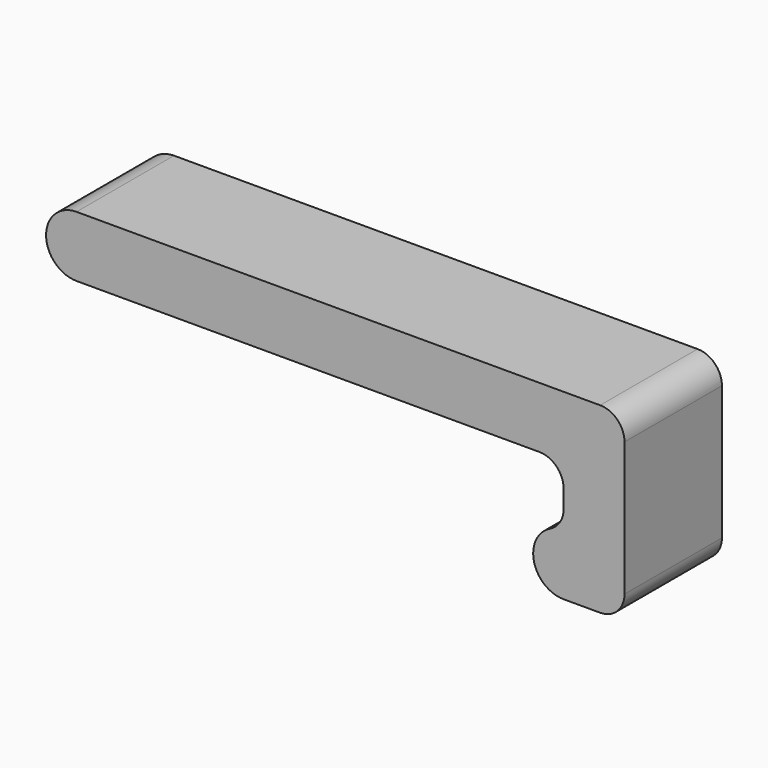
from build123d import *

# Parameters (mm, degrees)
F1_DEPTH = 20
F2_R     = 2.5
F3_DEPTH = 2
F4_R     = 0.99999


# Not quite as in the source:
# - a fillet or chamfer is up to 0.001 mm smaller than in the source, because OpenCascade refuses the exact size


with BuildPart() as f1:
    # F0 (on Front) → F1 (new body)
    with BuildSketch(Plane.XZ):
        with BuildLine():
            ThreePointArc((-42.5, 10), (-47.5, 5), (-42.5, 0))
            Line((-42.5, 0), (33.5, 0))
            ThreePointArc((33.5, 0), (36.3284271247, -1.1715728753), (37.5, -4))
            Line((37.5, -4), (37.5, -6.9377422517))
            ThreePointArc((37.5, -6.9377422517), (36.8993463424, -9.0459273585), (35.2777777778, -10.5209679176))
            ThreePointArc((35.2777777778, -10.5209679176), (32.6319839559, -16.1412360816), (37.5, -20))
            Line((37.5, -20), (43.5, -20))
            ThreePointArc((43.5, -20), (46.3284271247, -18.8284271247), (47.5, -16))
            Line((47.5, -16), (47.5, 6))
            ThreePointArc((47.5, 6), (46.3284271247, 8.8284271247), (43.5, 10))
            Line((43.5, 10), (-42.5, 10))
        make_face()
    extrude(amount=F1_DEPTH)

    # F2 (on face) → F3 (join)
    with BuildSketch(Plane(origin=(0, 0, 0), x_dir=(1, 0, 0), z_dir=(0, 0, -1))):
        with Locations((-23.5, 10)):
            Circle(F2_R)
        with Locations((23.5, 10)):
            Circle(F2_R)
    extrude(amount=F3_DEPTH)

    # F4 (radius 1 in the source; OpenCascade refuses exactly that, so slightly less here)
    f4_edges = [f1.edges().sort_by_distance(p)[0] for p in [
        (-26, -10, 0),
        (-26, -10, -2),
        (21, -10, 0),
        (21, -10, -2),
    ]]
    fillet(f4_edges, radius=F4_R)


solid = f1.part
